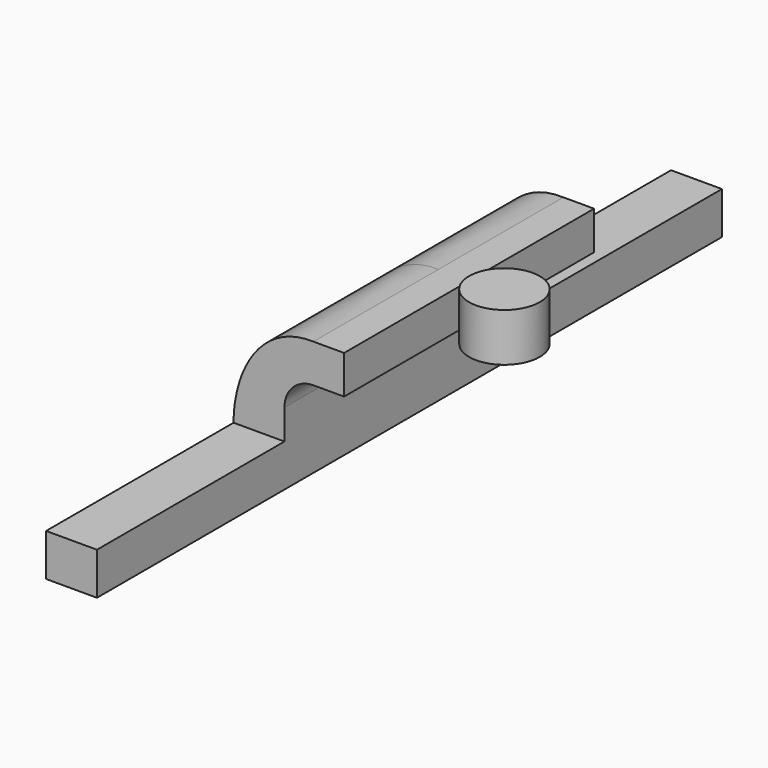
from build123d import *

# Parameters (mm, degrees)
F0_W     = 8.2724904759
F0_H     = 6.8799975622
F1_DEPTH = 63.5
F2_DEPTH = 25.4


with BuildPart() as f1:
    # F0 (on Front) → F1 (new body, symmetric)
    with BuildSketch(Plane.XZ):
        Rectangle(F0_W, F0_H)
    extrude(amount=F1_DEPTH, both=True)

    # F0 (on Front) → F2 (join, symmetric)
    with BuildSketch(Plane.XZ):
        with BuildLine():
            add(Edge.make_bspline(
                [(8.8344048709, 19.2660813623), (0.2333819866, 19.5338707417), (-4.1649181363, 11.0128456192), (-4.1362452379, 3.4399987811)],
                knots=[0, 0, 0, 0, 20.4622250528, 20.4622250528, 20.4622250528, 20.4622250528], degree=3))
            Line((-4.1362452379, 3.4399987811), (4.1362452379, 3.4399987811))
            Line((4.1362452379, 3.4399987811), (4.1362452379, 8.3213185052))
            ThreePointArc((4.1362452379, 8.3213185052), (5.5123043353, 11.6434190407), (8.8344048709, 13.0194781381))
            Line((8.8344048709, 13.0194781381), (13.8307970829, 13.0194781381))
            Line((13.8307970829, 13.0194781381), (13.8307970829, 16.8308063556))
            Line((13.8307970829, 16.8308063556), (13.8307970829, 19.2660813623))
            Line((13.8307970829, 19.2660813623), (8.8344048709, 19.2660813623))
        make_face()
    extrude(amount=F2_DEPTH, both=True)


with BuildPart() as f3:
    # F0 (on Front) → F3 (revolve)
    with BuildSketch(Plane.XZ):
        Polygon((19.5737686008, 19.9436039542), (19.5737686008, 19.2660813623), (19.5737686008, 17.6438695487), (19.5737686008, 16.0216577351), (19.5737686008, 16.0211566895), (19.5737686008, 13.0194781381), (19.5737686008, 12.099711516), (25.3167401188, 12.099711516), (25.3167401188, 19.9436039542), align=None)
    revolve(axis=Axis((19.5737686008, 0, 17.6438695487), (0, 0, 1)))


solid = Compound([f1.part, f3.part])
